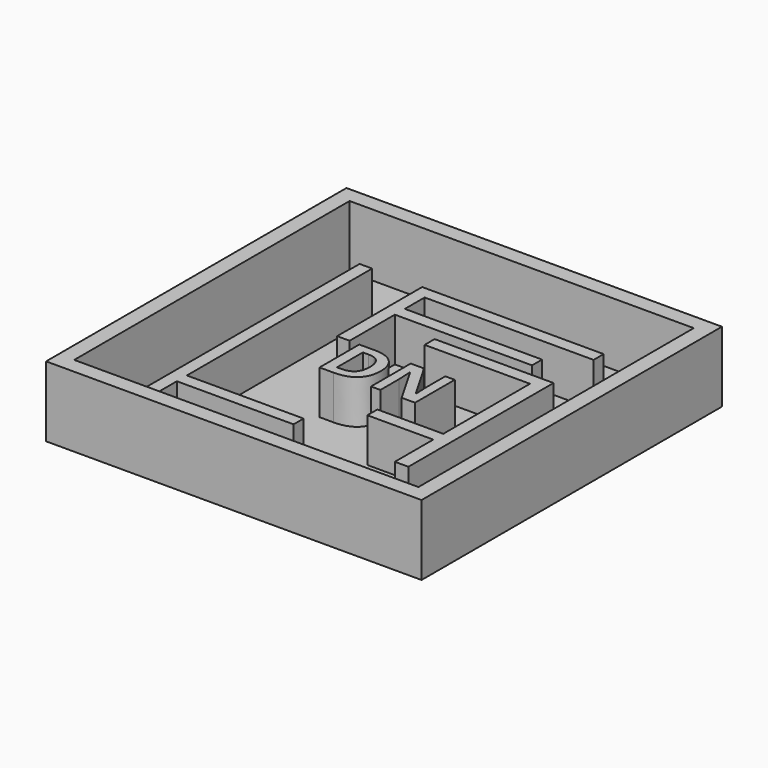
from build123d import *

# Parameters (mm, degrees)
F0_W         = 38.1
F0_H         = 38.1
F1_DEPTH     = 0.79375
F2_W         = 38.1
F2_H         = 38.1
F2_W_2       = 34.925
F2_H_2       = 34.925
F3_DEPTH     = 6.35
F4_W         = 1.27
F4_H         = 29.845
F5_DEPTH     = 4.445
F6_TEXT_SIZE = 7.0555555556
F7_DEPTH     = 4.445
F9_DEPTH     = 4.445
F11_DEPTH    = 4.445
F12_R        = 1.27
F13_DEPTH    = 0.396875
F14_W        = 13.9232961804
F14_H        = 1.27
F15_DEPTH    = 4.445
F16_R        = 1.27
F17_DEPTH    = 0.396875
F16_W        = 11.8422813427
F16_H        = 1.27
F18_DEPTH    = 4.445
F19_W        = 6.6881128465
F19_H        = 1.27
F20_DEPTH    = 4.445


# Not quite as in the source:
# - Text() gives the source's letters only with a copy of the font that has no kerning and outlines rounded to 1/6400 em; it was checked with that copy


with BuildPart() as f1:
    # F0 (on Top) → F1 (new body)
    with BuildSketch(Plane.XY):
        with Locations((0.2184137702, 2.9273987354)):
            Rectangle(F0_W, F0_H)
    extrude(amount=F1_DEPTH)

    # F2 (on face) → F3 (join)
    with BuildSketch(Plane.XY.offset(0.79375)):
        with Locations((0.2184137702, 2.9273987354)):
            Rectangle(F2_W, F2_H)
        with Locations((0.2184137702, 2.9273987354)):
            Rectangle(F2_W_2, F2_H_2, mode=Mode.SUBTRACT)
    extrude(amount=F3_DEPTH)

    # F4 (on face) → F5 (join)
    with BuildSketch(Plane.XY.offset(0.79375)):
        with Locations((-11.5290862298, 0.3873987354)):
            Rectangle(F4_W, F4_H)
    extrude(amount=F5_DEPTH)

    # F6 (on face) → F7 (join)
    with BuildSketch(Plane.XY.offset(0.79375)):
        with Locations((-4.1791123196, -0.5440522233)):
            Text('DN', F6_TEXT_SIZE, font='Open Sans', font_style=FontStyle.BOLD, text_align=(TextAlign.LEFT, TextAlign.BOTTOM))
    extrude(amount=F7_DEPTH)

    # F8 (on face) → F9 (join)
    with BuildSketch(Plane.XY.offset(0.79375)):
        Polygon((-5.8140862298, 15.3098987354), (-5.8140862298, 4.5224167482), (-4.5440862298, 4.5224167482), (-4.5440862298, 14.0324329375), (12.6009137702, 14.0324329375), (12.6009137702, 15.3098987354), align=None)
    extrude(amount=F9_DEPTH)

    # F10 (on face) → F11 (join)
    with BuildSketch(Plane.XY.offset(0.79375)):
        Polygon((12.6009137702, 8.9524329375), (0.5359137702, 8.9524329375), (0.5359137702, 7.6824329375), (11.2262522637, 7.6824329375), (11.2262522637, -9.4551012646), (12.6009137702, -9.4551012646), (12.6009137702, 7.6824329375), align=None)
    extrude(amount=F11_DEPTH)

    # F12 (on face) → F13 (cut)
    with BuildSketch(Plane.XY.offset(0.79375)):
        with Locations((-14.7040862298, -10.7251012646)):
            Circle(F12_R)
    extrude(amount=-F13_DEPTH, mode=Mode.SUBTRACT)

    # F14 (on face) → F15 (join)
    with BuildSketch(Plane.XY.offset(0.79375)):
        with Locations((2.4175618604, 10.8898253569)):
            Rectangle(F14_W, F14_H)
    extrude(amount=F15_DEPTH)

    # F16 (on face) → F17 (cut)
    with BuildSketch(Plane.XY.offset(0.79375)):
        with Locations((-7.6853204519, -11.9423987344)):
            Circle(F16_R)
    extrude(amount=-F17_DEPTH, mode=Mode.SUBTRACT)

    # F16 (on face) → F18 (join)
    with BuildSketch(Plane.XY.offset(0.79375)):
        with Locations((-4.9729455585, -8.8201012646)):
            Rectangle(F16_W, F16_H)
    extrude(amount=F18_DEPTH)

    # F19 (on face) → F20 (join)
    with BuildSketch(Plane.XY.offset(0.79375)):
        with Locations((7.8821958405, -3.94991873)):
            Rectangle(F19_W, F19_H)
    extrude(amount=F20_DEPTH)


solid = f1.part
